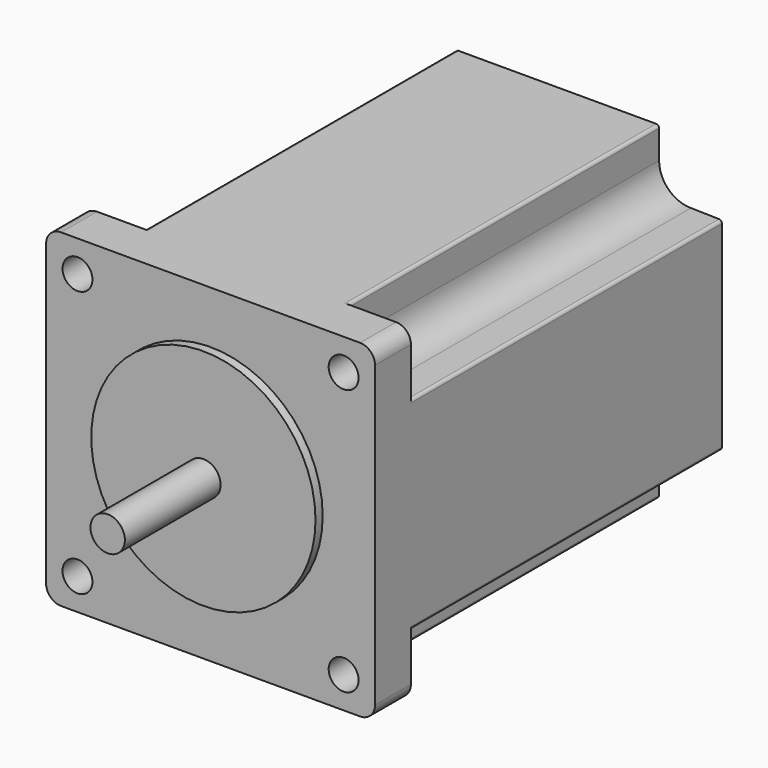
from build123d import *

# Parameters (mm, degrees)
F0_R     = 18.75
F1_DEPTH = 1.5
F0_R_2   = 2.5
F2_DEPTH = 7.5
F4_DEPTH = 65
F5_R     = 0.5
F6_R     = 2.875
F7_DEPTH = 20


with BuildPart() as f1:
    # F0 (on Front) → F1 (new body)
    with BuildSketch(Plane.XZ):
        Circle(F0_R)
    extrude(amount=F1_DEPTH)

    # F0 (on Front) → F2 (join)
    with BuildSketch(Plane.XZ):
        with BuildLine():
            Line((25, 27.5), (-25, 27.5))
            ThreePointArc((-25, 27.5), (-26.767766953, 26.767766953), (-27.5, 25))
            Line((-27.5, 25), (-27.5, -25))
            ThreePointArc((-27.5, -25), (-26.767766953, -26.767766953), (-25, -27.5))
            Line((-25, -27.5), (25, -27.5))
            ThreePointArc((25, -27.5), (26.767766953, -26.767766953), (27.5, -25))
            Line((27.5, -25), (27.5, 25))
            ThreePointArc((27.5, 25), (26.767766953, 26.767766953), (25, 27.5))
        make_face()
        with Locations((-22.25, -22.25)):
            Circle(F0_R_2, mode=Mode.SUBTRACT)
        with Locations((22.25, -22.25)):
            Circle(F0_R_2, mode=Mode.SUBTRACT)
        with Locations((-22.25, 22.25)):
            Circle(F0_R_2, mode=Mode.SUBTRACT)
        Circle(F0_R, mode=Mode.SUBTRACT)
        with Locations((22.25, 22.25)):
            Circle(F0_R_2, mode=Mode.SUBTRACT)
        Circle(F0_R)
    extrude(amount=-F2_DEPTH)

    # F3 (on face) → F4 (join)
    with BuildSketch(Plane(origin=(0, 7.5, 0), x_dir=(-1, 0, 0), z_dir=(0, 1, 0))):
        with BuildLine():
            Line((27.5, -17.0038467285), (27.5, 16.874561323))
            Line((27.5, 16.874561323), (22.1223071391, 17.0053998878))
            ThreePointArc((22.1223071391, 17.0053998878), (18.4928159277, 18.5869603521), (17.000002275, 22.253845591))
            Line((17.000002275, 22.253845591), (17.000002275, 27.5))
            Line((17.000002275, 27.5), (-17.000002275, 27.5))
            Line((-17.000002275, 27.5), (-17.000002275, 22.253845591))
            ThreePointArc((-17.000002275, 22.253845591), (-18.5623015375, 18.5132408344), (-22.3232260335, 17.0005115574))
            Line((-22.3232260335, 17.0005115574), (-27.5, 16.874561323))
            Line((-27.5, 16.874561323), (-27.5, -17.0038467285))
            Line((-27.5, -17.0038467285), (-22.4509152226, -17.0038467285))
            ThreePointArc((-22.4509152226, -17.0038467285), (-18.6080321838, -18.4686563976), (-17.000002275, -22.253845591))
            Line((-17.000002275, -22.253845591), (-17.000002275, -27.5))
            Line((-17.000002275, -27.5), (17.000002275, -27.5))
            Line((17.000002275, -27.5), (17.000002275, -22.253845591))
            ThreePointArc((17.000002275, -22.253845591), (18.5376913406, -18.5415357941), (22.2500011375, -17.0038467285))
            Line((22.2500011375, -17.0038467285), (27.5, -17.0038467285))
        make_face()
    extrude(amount=F4_DEPTH)

    # F5
    f5_edges = [f1.edges().sort_by_distance(p)[0] for p in [
        (17.000002, 40, 27.5),
        (-17.000002, 40, 27.5),
        (27.5, 40, -17.003847),
        (27.5, 40, 16.874561),
        (-27.5, 40, 16.874561),
        (-27.5, 40, -17.003847),
        (-17.000002, 40, -27.5),
        (17.000002, 40, -27.5),
    ]]
    fillet(f5_edges, radius=F5_R)

    # F6 (on face) → F7 (join)
    with BuildSketch(Plane.XZ.offset(1.5)):
        Circle(F6_R)
    extrude(amount=F7_DEPTH)


solid = f1.part
